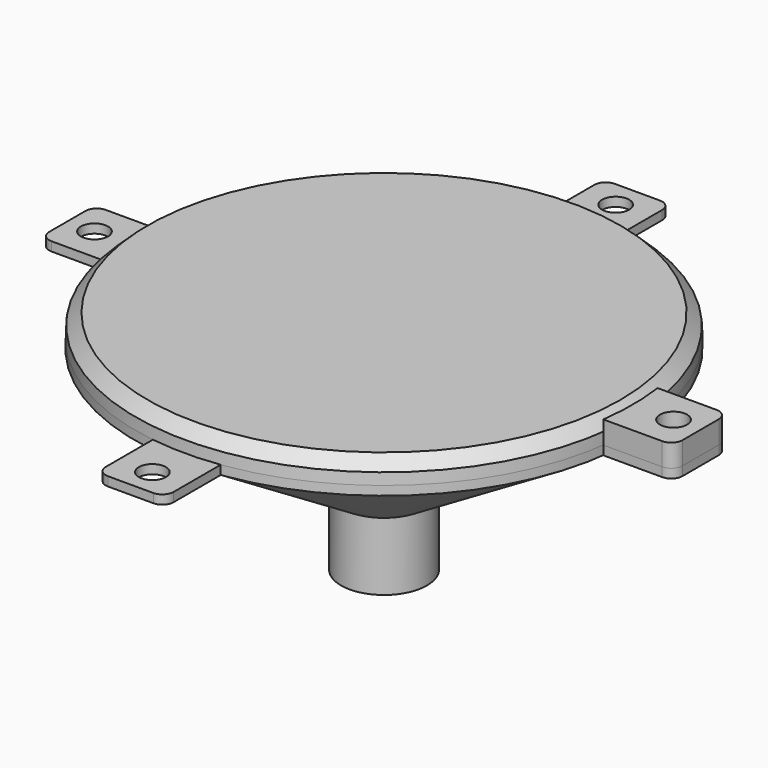
from build123d import *

# Parameters (mm, degrees)
F2_R     = 6
F3_DEPTH = 4
F4_COUNT = 4
F8_R     = 110
F9_DEPTH = 10
F9_TAPER = 3
F6_R     = 6
F7_DEPTH = 10


# Not quite as in the source:
# - a fillet or chamfer that OpenCascade refuses, or shapes differently, is made with other operations: its cross-section is extruded or revolved along the edge and cut away or added


with BuildPart() as f1:
    # F0 (on Front) → F1 (revolve)
    with BuildSketch(Plane.XZ):
        Polygon((19, 30), (110, 86), (110, 90), (106, 90), (19, 36.4615384615), (15, 36.4615384615), (15, 0), (19, 0), align=None)
    revolve(axis=Axis((0, 0, 18.2307692308), (0, 0, 1)))


with BuildPart() as f3:
    # F2 (on face) → F3 (new body)
    with BuildSketch(Plane.XY.offset(90)):
        with BuildLine():
            ThreePointArc((108.9724735885, 15), (110, 0), (108.9724735885, -15))
            Line((108.9724735885, -15), (135, -15))
            ThreePointArc((135, -15), (138.5355339059, -13.5355339059), (140, -10))
            Line((140, -10), (140, 10))
            ThreePointArc((140, 10), (138.5355339059, 13.5355339059), (135, 15))
            Line((135, 15), (108.9724735885, 15))
        make_face()
        with Locations((128, 0)):
            Circle(F2_R, mode=Mode.SUBTRACT)
    extrude(amount=-F3_DEPTH)


with BuildPart() as f4_1:
    # F4: instance of F3
    add(f3.part.rotate(Axis((0, 0, 36.4615384615), (0, 0, -1)), 1 * 360 / F4_COUNT))


with BuildPart() as f4_2:
    # F4: instance of F3
    add(f3.part.rotate(Axis((0, 0, 36.4615384615), (0, 0, -1)), 2 * 360 / F4_COUNT))


with BuildPart() as f4_3:
    # F4: instance of F3
    add(f3.part.rotate(Axis((0, 0, 36.4615384615), (0, 0, -1)), 3 * 360 / F4_COUNT))


with BuildPart() as f9:
    # F8 (on face) → F9 (new body)
    with BuildSketch(Plane.XY.offset(90)):
        Circle(F8_R)
    extrude(amount=F9_DEPTH, taper=F9_TAPER)

    # F5: chamfer of 5 on 1 edges, made by hand

    # F5_s1 → F5_t2 (revolve, cut)
    with BuildSketch(Plane.XZ):
        Polygon((109.7376019884, 95.0068523262), (104.4759222072, 100), (109.4759222072, 100), align=None)
    revolve(axis=Axis((0, 0, 100), (0, 0, -1)), mode=Mode.SUBTRACT)


with BuildPart() as f7:
    # F6 (on face) → F7 (new body)
    with BuildSketch(Plane.XY.offset(90)):
        with BuildLine():
            Line((108.9724735885, -15), (135, -15))
            ThreePointArc((135, -15), (138.5355339059, -13.5355339059), (140, -10))
            Line((140, -10), (140, 10))
            ThreePointArc((140, 10), (138.5355339059, 13.5355339059), (135, 15))
            Line((135, 15), (108.9724735885, 15))
            ThreePointArc((108.9724735885, 15), (110, 0), (108.9724735885, -15))
        make_face()
        with Locations((128, 0)):
            Circle(F6_R, mode=Mode.SUBTRACT)
    extrude(amount=F7_DEPTH)


solid = Compound([f1.part, f3.part, f4_1.part, f4_2.part, f4_3.part, f9.part, f7.part])
